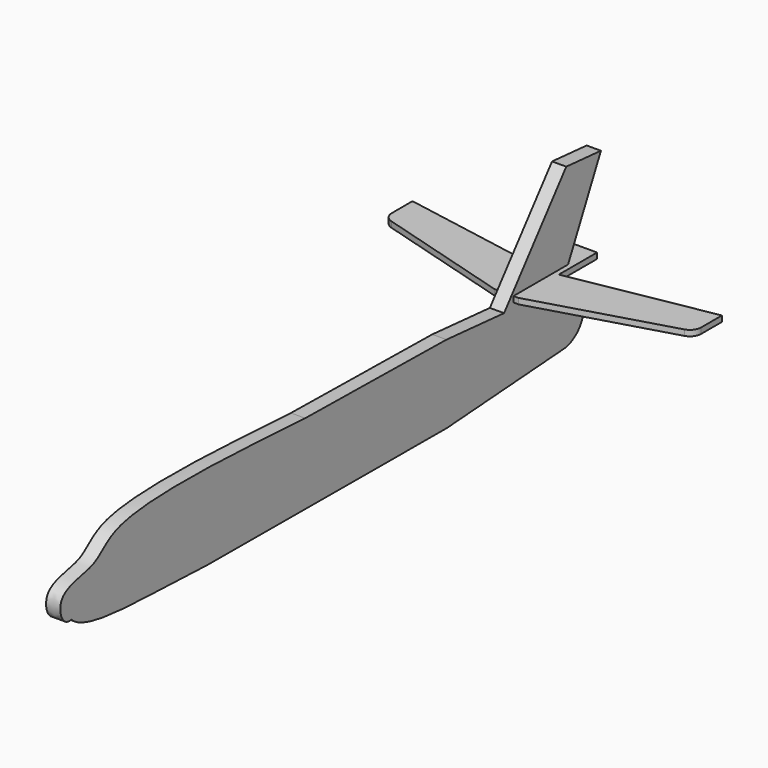
from build123d import *

# Parameters (mm, degrees)
F1_DEPTH = 6.35
F2_W     = 43.8992977142
F2_H     = 2.5489926338
F3_DEPTH = 132.08
F5_DEPTH = 25.4


# Not quite as in the source:
# - a feature names something its author has since deleted; it is built from what else it names


with BuildPart() as f1:
    # F0 (on Right) → F1 (new body)
    with BuildSketch(Plane.YZ):
        with BuildLine():
            Line((76.3076053803, 30.0652621201), (-2.577113572, 31.2436707318))
            add(Edge.make_bspline(
                [(-2.577113572, 31.2436707318), (-18.9517831163, 31.8808788266), (-110.584283844, 39.3805456931), (-117.2445348924, 19.5506491484), (-143.4980605313, 19.8314466417), (-138.213646076, 4.0164198283), (-133.0822259188, 5.1160147414)],
                knots=[0, 0, 0, 0, 0.4568495448, 0.6533081411, 0.8493490225, 1, 1, 1, 1], degree=3))
            add(Edge.make_bspline(
                [(-57.4250192094, -4.2738611867), (-92.646561563, -2.3575690575), (-123.9624172449, -4.0037976578), (-133.0822259188, 5.1160147414)],
                knots=[0, 0, 0, 0, 76.2376724265, 76.2376724265, 76.2376724265, 76.2376724265], degree=3))
            Line((-57.4250192094, -4.2738611867), (76.3076053803, -4.8074758588))
            Line((76.3076053803, -4.8074758588), (140.6258685644, -0.2679234478))
            ThreePointArc((140.6258685644, -0.2679234478), (152.6195542591, 8.6888150074), (147.4371024588, 22.732100009))
            Line((147.4371024588, 22.732100009), (140.6258685644, 24.7491808721))
            Line((140.6258685644, 24.7491808721), (162.5416169533, 69.2932593767))
            Line((162.5416169533, 69.2932593767), (143.1825459003, 70.8933398128))
            Line((143.1825459003, 70.8933398128), (108.4667369723, 27.4072214961))
            Line((108.4667369723, 27.4072214961), (76.3076053803, 30.0652621201))
        make_face()
    extrude(amount=F1_DEPTH)


with BuildPart() as f3:
    # F2 (on Right) → F3 (new body, symmetric)
    with BuildSketch(Plane.YZ):
        with Locations((135.6572210789, 30.7295061648)):
            Rectangle(F2_W, F2_H)
    extrude(amount=F3_DEPTH, both=True)

    # F4 (on face) → F5 (cut)
    with BuildSketch(Plane.XY.offset(32.0040024817)):
        with BuildLine():
            Line((68.6163709771, 131.2541425074), (8.5697518662, 113.7075722218))
            Line((8.5697518662, 113.7075722218), (11.151721701, 106.6866666079))
            Line((11.151721701, 106.6866666079), (138.4570300579, 103.6873310804))
            Line((138.4570300579, 103.6873310804), (142.1228945255, 164.6739095449))
            Line((142.1228945255, 164.6739095449), (8.5697518662, 160.3934181468))
            Line((8.5697518662, 160.3934181468), (8.5697518662, 136.2849026918))
            Line((8.5697518662, 136.2849026918), (72.2715035081, 147.6867645979))
            Line((72.2715035081, 147.6867645979), (72.2715035081, 136.1302221516))
            ThreePointArc((72.2715035081, 136.1302221516), (71.256274519, 133.0832504371), (68.6163709771, 131.2541425074))
        make_face()
        with BuildLine():
            Line((-65.9215035081, 147.6867645979), (-2.2197518662, 136.2849026918))
            Line((-2.2197518662, 136.2849026918), (-2.2197518662, 160.3934181468))
            Line((-2.2197518662, 160.3934181468), (-135.7728945255, 164.6739095449))
            Line((-135.7728945255, 164.6739095449), (-132.1070300579, 103.6873310804))
            Line((-132.1070300579, 103.6873310804), (-4.801721701, 106.6866666079))
            Line((-4.801721701, 106.6866666079), (-2.2197518662, 113.7075722218))
            Line((-2.2197518662, 113.7075722218), (-62.2663709771, 131.2541425074))
            ThreePointArc((-62.2663709771, 131.2541425074), (-64.906274519, 133.0832504371), (-65.9215035081, 136.1302221516))
            Line((-65.9215035081, 136.1302221516), (-65.9215035081, 147.6867645979))
        make_face()
    extrude(amount=-F5_DEPTH, mode=Mode.SUBTRACT)


solid = Compound([f1.part, f3.part])
